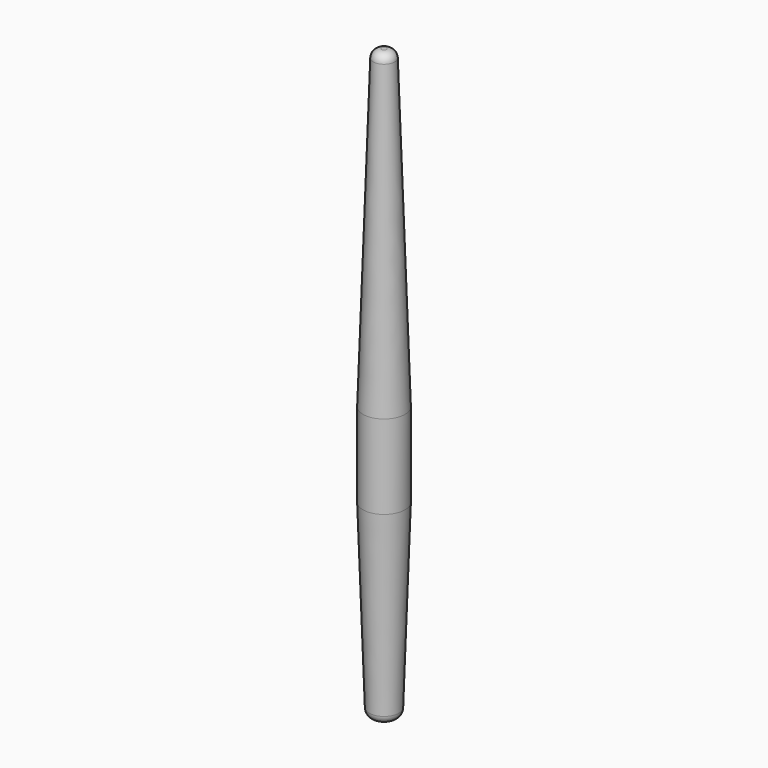
from build123d import *

# Parameters (mm, degrees)
F2_R      = 5
F0_R      = 3.5
F4_R      = 2
F3_FACE_R = 5
F6_R      = 5
F7_FACE_R = 5
F9_R      = 2.5
F11_R     = 2


with BuildPart() as f3:
    # F2 (on offset) → F3 section 0
    with BuildSketch(Plane.XY.offset(45)):
        Circle(F2_R)
    # F0 (on Top) → F3 section 1
    with BuildSketch(Plane.XY):
        Circle(F0_R)
    loft()

    # F4
    f4_edges = [f3.edges().sort_by_distance(p)[0] for p in [
        (-3.5, 0, 0),
    ]]
    fillet(f4_edges, radius=F4_R)

    # F3_face (on face) → F7 section 0
    with BuildSketch(Plane.XY.offset(45)):
        Circle(F3_FACE_R)
    # F6 (on offset) → F7 section 1
    with BuildSketch(Plane.XY.offset(65)):
        Circle(F6_R)
    loft()

    # F7_face (on face) → F10 section 0
    with BuildSketch(Plane.XY.offset(65)):
        Circle(F7_FACE_R)
    # F9 (on offset) → F10 section 1
    with BuildSketch(Plane.XY.offset(140)):
        Circle(F9_R)
    loft()

    # F11
    f11_edges = [f3.edges().sort_by_distance(p)[0] for p in [
        (-2.5, 0, 140),
    ]]
    fillet(f11_edges, radius=F11_R)


solid = f3.part
